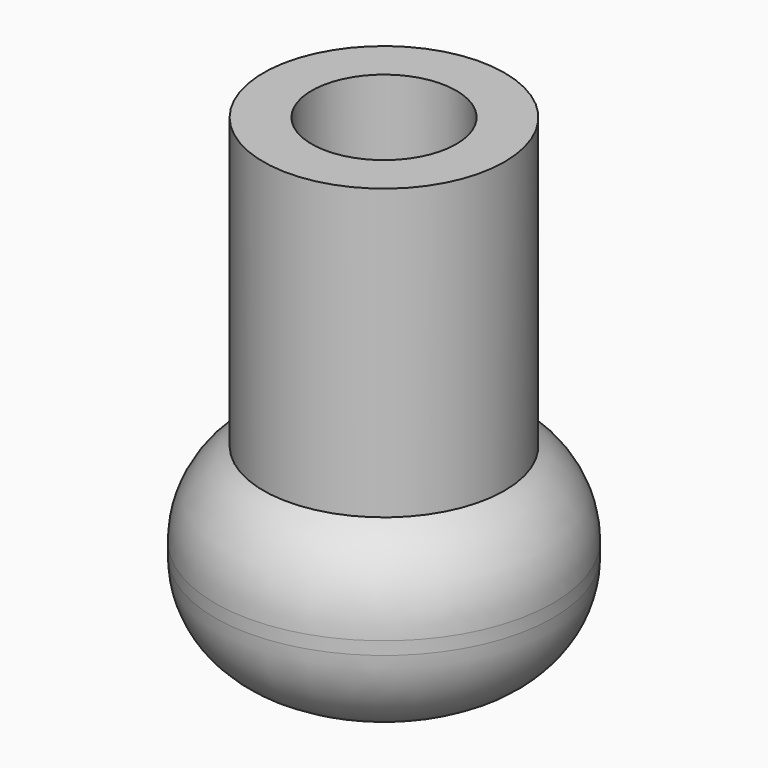
from build123d import *

# Parameters (mm, degrees)
F0_R     = 2.5
F0_R_2   = 1.5
F1_DEPTH = 6
F2_DEPTH = 7
F3_R     = 3.5
F3_R_2   = 2.5
F3_R_3   = 1.5
F4_DEPTH = 4


# Not quite as in the source:
# - a fillet or chamfer that OpenCascade refuses, or shapes differently, is made with other operations: its cross-section is extruded or revolved along the edge and cut away or added


with BuildPart() as f1:
    # F0 (on Top) → F1 (new body)
    with BuildSketch(Plane.XY):
        Circle(F0_R)
        Circle(F0_R_2, mode=Mode.SUBTRACT)
    extrude(amount=-F1_DEPTH)

    # F0 (on Top) → F2 (cut)
    with BuildSketch(Plane.XY):
        Circle(F0_R_2)
    extrude(amount=-F2_DEPTH, mode=Mode.SUBTRACT)

    # F3 (on face) → F4 (join)
    with BuildSketch(Plane(origin=(0, 0, -6), x_dir=(1, 0, 0), z_dir=(0, 0, -1))):
        Circle(F3_R)
        Circle(F3_R_2, mode=Mode.SUBTRACT)
        Circle(F3_R_2)
        Circle(F3_R_3, mode=Mode.SUBTRACT)
        Circle(F3_R_3)
    extrude(amount=F4_DEPTH)

    # F5: fillet of radius 2 on 2 edges, made by hand

    # F5_s1 → F5_t2 (revolve, cut)
    with BuildSketch(Plane.XZ):
        with BuildLine():
            ThreePointArc((3.5, -8), (2.9142135624, -9.4142135624), (1.5, -10))
            Line((1.5, -10), (3.5, -10))
            Line((3.5, -10), (3.5, -8))
        make_face()
    revolve(axis=Axis((0, 0, -10), (0, 0, -1)), mode=Mode.SUBTRACT)

    # F5_s3 → F5_t4 (revolve, cut)
    with BuildSketch(Plane.XZ):
        with BuildLine():
            ThreePointArc((3.5, -7.7320508076), (3.2320508076, -6.7320508076), (2.5, -6))
            Line((2.5, -6), (3.5, -6))
            Line((3.5, -6), (3.5, -7.7320508076))
        make_face()
    revolve(axis=Axis((0, 0, -6), (0, 0, -1)), mode=Mode.SUBTRACT)


solid = f1.part
